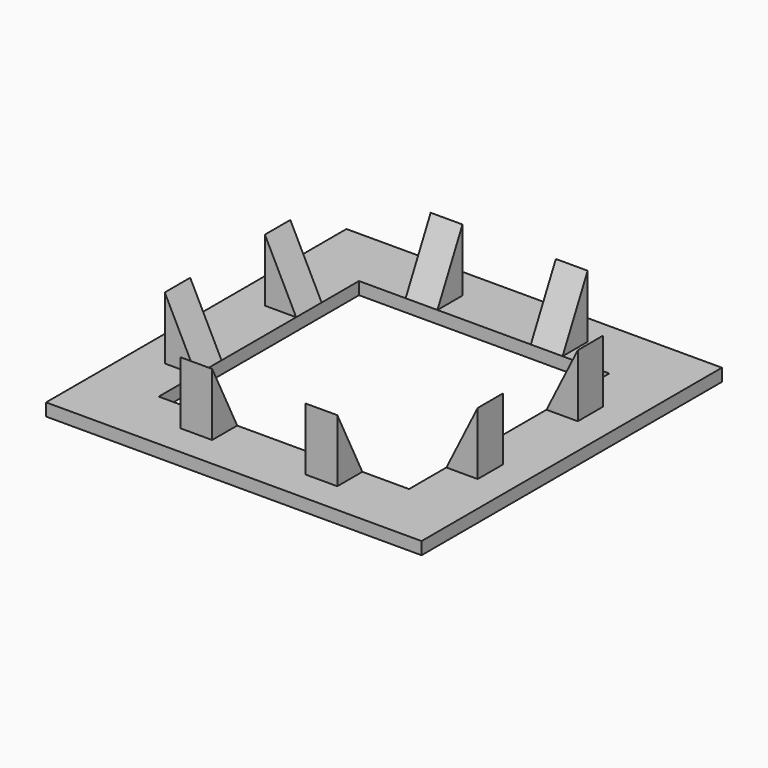
from build123d import *

# Parameters (mm, degrees)
F0_W      = 600
F0_H      = 600
F1_DEPTH  = 20
F2_W      = 50
F2_H      = 20
F3_W      = 50
F3_H      = 20
F8_DEPTH  = 50.8
F4_W      = 50
F4_H      = 20
F5_W      = 50
F5_H      = 20
F11_DEPTH = 50.8
F6_W      = 50
F6_H      = 20
F7_W      = 50
F7_H      = 20
F12_DEPTH = 50.8
F9_W      = 50
F9_H      = 20
F10_W     = 50
F10_H     = 20
F13_DEPTH = 50.8


# Not quite as in the source:
# - a feature names something its author has since deleted; it is built from what else it names


with BuildPart() as f1:
    # F0 (on Top) → F1 (new body)
    with BuildSketch(Plane.XY):
        with Locations((-57.8414618969, -13.7785196304)):
            Rectangle(F0_W, F0_H)
        Polygon((-257.8414618969, 111.6214803696), (-257.8414618969, 186.2214803696), (-183.2414618969, 186.2214803696), (-183.2414618969, 236.2214803696), (-157.8414618969, 236.2214803696), (-132.4414618969, 236.2214803696), (-132.4414618969, 186.2214803696), (16.7585381031, 186.2214803696), (16.7585381031, 236.2214803696), (67.5585381031, 236.2214803696), (67.5585381031, 186.2214803696), (142.1585381031, 186.2214803696), (142.1585381031, 111.6214803696), (192.1585381031, 111.6214803696), (192.1585381031, 60.8214803696), (142.1585381031, 60.8214803696), (142.1585381031, -88.3785196304), (192.1585381031, -88.3785196304), (192.1585381031, -139.1785196304), (142.1585381031, -139.1785196304), (142.1585381031, -213.7785196304), (67.5585381031, -213.7785196304), (67.5585381031, -263.7785196304), (16.7585381031, -263.7785196304), (16.7585381031, -213.7785196304), (-132.4414618969, -213.7785196304), (-132.4414618969, -263.7785196304), (-183.2414618969, -263.7785196304), (-183.2414618969, -213.7785196304), (-257.8414618969, -213.7785196304), (-257.8414618969, -139.1785196304), (-307.8414618969, -139.1785196304), (-307.8414618969, -88.3785196304), (-257.8414618969, -88.3785196304), (-257.8414618969, -13.7785196304), (-257.8414618969, 60.8214803696), (-307.8414618969, 60.8214803696), (-307.8414618969, 111.6214803696), align=None, mode=Mode.SUBTRACT)
    extrude(amount=F1_DEPTH)

    # F2 (on face) + F3 (on face) → F8 (join)
    with BuildSketch(Plane.XZ.offset(88.3785196304)):
        Polygon((-307.8414618969, 20), (-257.8414618969, 20), (-307.8414618969, 120), align=None)
        with Locations((-282.8414618969, 10)):
            Rectangle(F2_W, F2_H)
    with BuildSketch(Plane.XZ.offset(-111.6214803696)):
        Polygon((-307.8414618969, 20), (-257.8414618969, 20), (-307.8414618969, 120), align=None)
        with Locations((-282.8414618969, 10)):
            Rectangle(F3_W, F3_H)
    extrude(amount=F8_DEPTH)

    # F4 (on face) + F5 (on face) → F11 (join)
    with BuildSketch(Plane(origin=(-132.4414618969, 0, 0), x_dir=(0, -1, 0), z_dir=(-1, 0, 0))):
        Polygon((-236.2214803696, 20), (-186.2214803696, 20), (-236.2214803696, 120), align=None)
        with Locations((-211.2214803696, 10)):
            Rectangle(F4_W, F4_H)
    with BuildSketch(Plane(origin=(67.5585381031, 0, 0), x_dir=(0, -1, 0), z_dir=(-1, 0, 0))):
        with Locations((-211.2214803696, 10)):
            Rectangle(F5_W, F5_H)
        Polygon((-236.2214803696, 20), (-186.2214803696, 20), (-236.2214803696, 120), align=None)
    extrude(amount=F11_DEPTH)

    # F6 (on face) + F7 (on face) → F12 (join)
    with BuildSketch(Plane(origin=(0, 60.8214803696, 0), x_dir=(-1, 0, 0), z_dir=(0, 1, 0))):
        with Locations((-167.1585381031, 10)):
            Rectangle(F6_W, F6_H)
        Polygon((-192.1585381031, 20), (-142.1585381031, 20), (-192.1585381031, 120), align=None)
    with BuildSketch(Plane(origin=(0, -139.1785196304, 0), x_dir=(-1, 0, 0), z_dir=(0, 1, 0))):
        with Locations((-167.1585381031, 10)):
            Rectangle(F7_W, F7_H)
        Polygon((-192.1585381031, 20), (-142.1585381031, 20), (-192.1585381031, 120), align=None)
    extrude(amount=F12_DEPTH)

    # F9 (on face) + F10 (on face) → F13 (join)
    with BuildSketch(Plane.YZ.offset(16.7585381031)):
        with Locations((-238.7785196304, 10)):
            Rectangle(F9_W, F9_H)
        Polygon((-263.7785196304, 20), (-213.7785196304, 20), (-263.7785196304, 120), align=None)
    with BuildSketch(Plane.YZ.offset(-183.2414618969)):
        with Locations((-238.7785196304, 10)):
            Rectangle(F10_W, F10_H)
        Polygon((-263.7785196304, 20), (-213.7785196304, 20), (-263.7785196304, 120), align=None)
    extrude(amount=F13_DEPTH)


solid = f1.part
